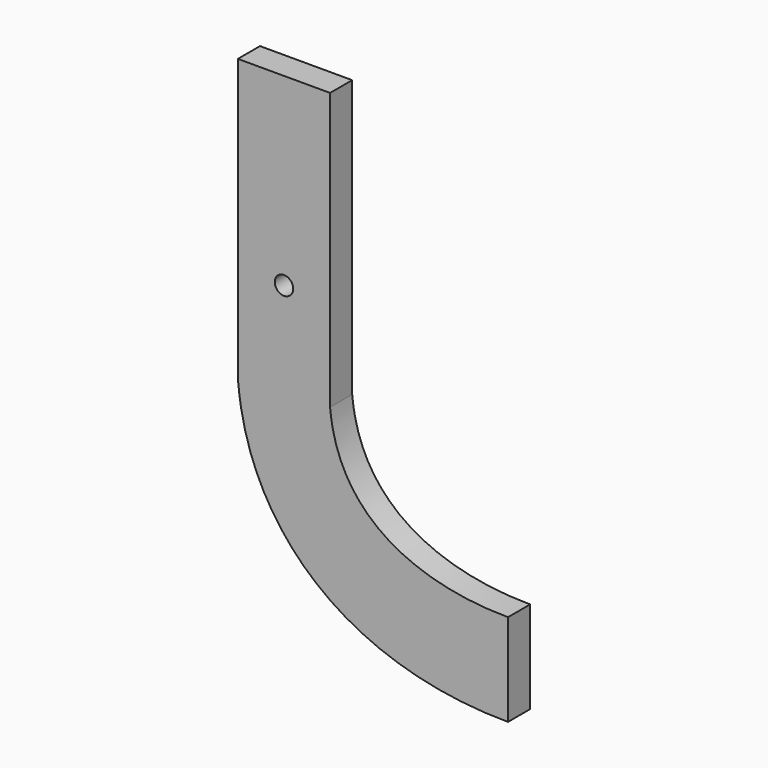
from build123d import *

# Parameters (mm, degrees)
F0_W     = 25.4
F0_H     = 76.2
F1_DEPTH = 7.62
F3_D     = 5.08


# Not quite as in the source:
# - the dataset's text gives a spline's control points without its knots; the knots are read off the source's solid


with BuildPart() as f1:
    # F0 (on Front) → F1 (new body)
    with BuildSketch(Plane.XZ):
        with BuildLine():
            Line((40.3294241467, -40.2762308451), (40.3294241467, -14.8762308451))
            add(Edge.make_bspline(
                [(40.3294241467, -14.8762308451), (21.5610041973, -14.8762308451), (-6.0386634815, -8.9048186666), (-8.6821928732, 20.1097459238)],
                knots=[0, 0, 0, 0, 60.217581929, 60.217581929, 60.217581929, 60.217581929], degree=3))
            Line((-8.6821928732, 20.1097459238), (-34.0821928732, 20.1097459238))
            Line((-34.0821928732, 20.1097459238), (-33.9774206207, 17.805086903))
            add(Edge.make_bspline(
                [(40.3294241467, -40.2762308451), (37.3099271571, -40.2762308451), (30.9115899013, -40.0382676619), (20.4384008636, -38.6684521368), (11.1591942082, -36.3483735395), (3.5451147785, -33.5001668079), (-2.2049298125, -30.7771521382), (-7.916216422, -27.3725582588), (-13.4738421139, -23.1950198102), (-18.7206219083, -18.1785503269), (-23.4642827177, -12.3091997018), (-27.5057889038, -5.6450934219), (-30.6818257575, 1.6886932692), (-32.898503265, 9.5359182195), (-33.7233931846, 15.0169599868), (-33.9774206207, 17.805086903)],
                knots=[0, 0, 0, 0, 0.125, 0.25, 0.375, 0.4375, 0.5, 0.5625, 0.625, 0.6875, 0.75, 0.8125, 0.875, 0.9375, 1, 1, 1, 1], degree=3))
        make_face()
        with Locations((-21.3821928732, 58.2097459238)):
            Rectangle(F0_W, F0_H)
    extrude(amount=F1_DEPTH)

    # F3 (through all)
    with Locations(Plane.XZ.offset(7.62)):
        with Locations((-21.3821928732, 45.5097459238)):
            Hole(F3_D / 2)


solid = f1.part
